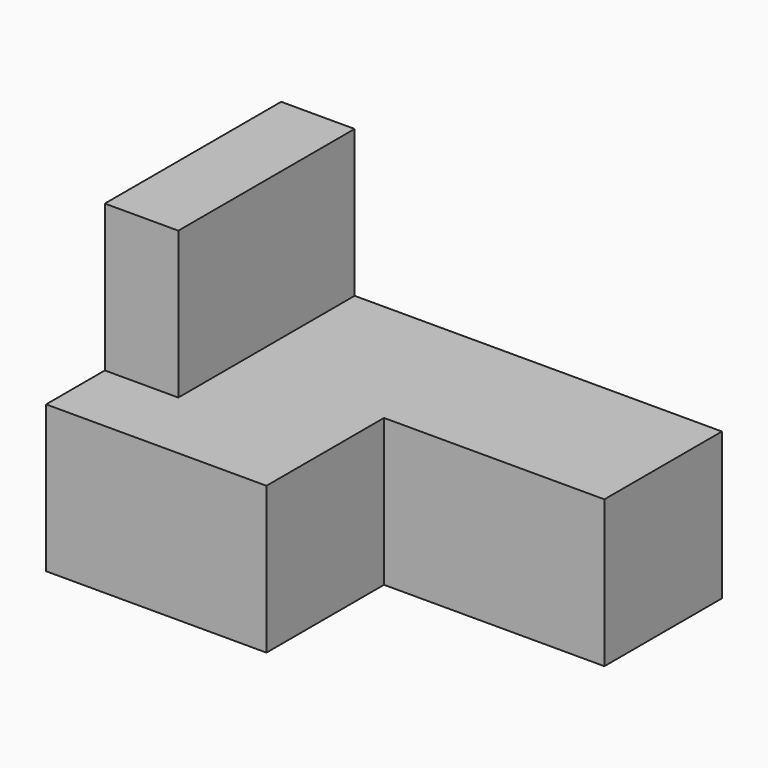
from build123d import *

# Parameters (mm, degrees)
F0_W     = 38.1
F0_H     = 12.7
F1_DEPTH = 12.7
F2_W     = 19.05
F2_H     = 12.7
F3_DEPTH = 12.701
F4_W     = 6.35
F4_H     = 12.7
F5_DEPTH = 12.7
F6_W     = 6.35
F6_H     = 6.35
F7_DEPTH = 25.401


with BuildPart() as f1:
    # F0 (on Front) → F1 (new body, symmetric)
    with BuildSketch(Plane.XZ):
        with Locations((19.05, 6.35)):
            Rectangle(F0_W, F0_H)
    extrude(amount=F1_DEPTH, both=True)

    # F2 (on Top) → F3 (cut, through all)
    with BuildSketch(Plane.XY):
        with Locations((28.575, -6.35)):
            Rectangle(F2_W, F2_H)
    extrude(amount=F3_DEPTH, mode=Mode.SUBTRACT)


with BuildPart() as f5:
    # F4 (on Front) → F5 (new body, symmetric)
    with BuildSketch(Plane.XZ):
        with Locations((3.175, 19.05)):
            Rectangle(F4_W, F4_H)
    extrude(amount=F5_DEPTH, both=True)

    # F6 (on Top) → F7 (cut, through all)
    with BuildSketch(Plane.XY):
        with Locations((3.175, -9.525)):
            Rectangle(F6_W, F6_H)
    extrude(amount=F7_DEPTH, mode=Mode.SUBTRACT)


solid = Compound([f1.part, f5.part])
